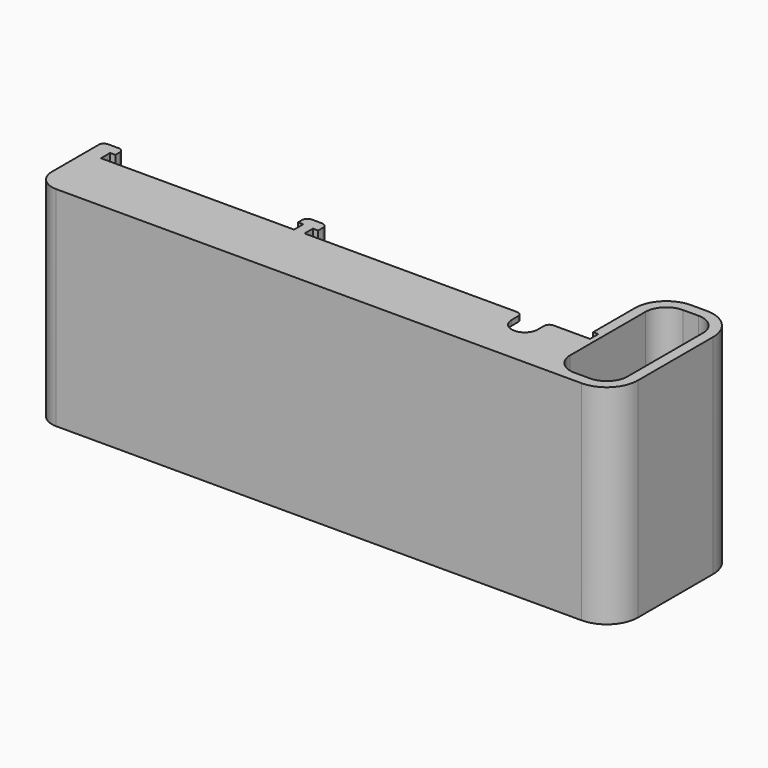
from build123d import *

# Parameters (mm, degrees)
F0_W     = 2
F0_H     = 8
F0_W_2   = 35
F0_H_2   = 10
F1_DEPTH = 40
F2_DEPTH = 39
F3_R     = 4
F4_R     = 0.99999
F5_R     = 6


# Not quite as in the source:
# - a fillet or chamfer is up to 0.001 mm smaller than in the source, because OpenCascade refuses the exact size


with BuildPart() as f1:
    # F0 (on Top) → F1 (new body)
    with BuildSketch(Plane.XY):
        Polygon((40.35, -15), (55.35, -15), (55.35, 15), (40.35, 15), (40.35, 1.2), (40.35, -1), (41.35, -1), (41.35, -3), (40.35, -3), (40.35, -13), align=None)
        Polygon((42.35, -13), (42.35, 1.2), (42.35, 13), (53.35, 13), (53.35, -13), align=None, mode=Mode.SUBTRACT)
        Polygon((-55.35, -15), (40.35, -15), (40.35, -13), (1.15, -13), (-0.85, -13), (-12.35, -13), (-16.35, -13), (-51.35, -13), (-55.35, -13), align=None)
        Polygon((-12.35, -1), (-12.35, 1.2), (-16.35, 1.2), (-16.35, -0.8), (-15.35, -0.8), (-15.35, -3), (-16.35, -3), (-16.35, -13), (-12.35, -13), (-12.35, -3), (-13.35, -3), (-13.35, -1), align=None)
        Polygon((-55.35, 1.2), (-55.35, -13), (-51.35, -13), (-51.35, -3), (-52.35, -3), (-52.35, -0.8), (-51.35, -0.8), (-51.35, 1.2), align=None)
        with Locations((0.15, -9)):
            Rectangle(F0_W, F0_H)
        with Locations((-33.85, -8)):
            Rectangle(F0_W_2, F0_H_2)
        with BuildLine():
            Line((1.15, -13), (40.35, -13))
            Line((40.35, -13), (40.35, -3))
            Line((40.35, -3), (33.35, -3))
            Line((33.35, -3), (33.35, -5.5))
            ThreePointArc((33.35, -5.5), (30.85, -8), (28.35, -5.5))
            Line((28.35, -5.5), (28.35, -3))
            Line((28.35, -3), (-12.35, -3))
            Line((-12.35, -3), (-12.35, -13))
            Line((-12.35, -13), (-0.85, -13))
            Line((-0.85, -13), (-0.85, -5))
            Line((-0.85, -5), (1.15, -5))
            Line((1.15, -5), (1.15, -13))
        make_face()
    extrude(amount=F1_DEPTH)

    # F0 (on Top) → F2 (cut)
    with BuildSketch(Plane.XY):
        with Locations((-33.85, -8)):
            Rectangle(F0_W_2, F0_H_2)
        with BuildLine():
            Line((1.15, -13), (40.35, -13))
            Line((40.35, -13), (40.35, -3))
            Line((40.35, -3), (33.35, -3))
            Line((33.35, -3), (33.35, -5.5))
            ThreePointArc((33.35, -5.5), (30.85, -8), (28.35, -5.5))
            Line((28.35, -5.5), (28.35, -3))
            Line((28.35, -3), (-12.35, -3))
            Line((-12.35, -3), (-12.35, -13))
            Line((-12.35, -13), (-0.85, -13))
            Line((-0.85, -13), (-0.85, -5))
            Line((-0.85, -5), (1.15, -5))
            Line((1.15, -5), (1.15, -13))
        make_face()
    extrude(amount=F2_DEPTH, mode=Mode.SUBTRACT)

    # F3
    f3_edges = [f1.edges().sort_by_distance(p)[0] for p in [
        (42.35, -13, 20),
        (53.35, -13, 20),
        (53.35, 13, 20),
        (42.35, 13, 20),
        (-55.35, -15, 20),
    ]]
    fillet(f3_edges, radius=F3_R)

    # F4 (radius 1 in the source; OpenCascade refuses exactly that, so slightly less here)
    f4_edges = [f1.edges().sort_by_distance(p)[0] for p in [
        (40.35, -13, 19.5),
        (-0.85, -13, 19.5),
        (-0.85, -5, 19.5),
        (-16.35, -13, 19.5),
        (-16.35, 1.2, 20),
        (-12.35, 1.2, 20),
        (-55.35, 1.2, 20),
        (-51.35, 1.2, 20),
        (-51.35, -13, 19.5),
        (1.15, -5, 19.5),
        (1.15, -13, 19.5),
        (-12.35, -13, 19.5),
        (33.35, -3, 39.5),
        (28.35, -3, 39.5),
    ]]
    fillet(f4_edges, radius=F4_R)

    # F5
    f5_edges = [f1.edges().sort_by_distance(p)[0] for p in [
        (40.35, 15, 20),
        (55.35, 15, 20),
        (55.35, -15, 20),
    ]]
    fillet(f5_edges, radius=F5_R)


solid = f1.part
